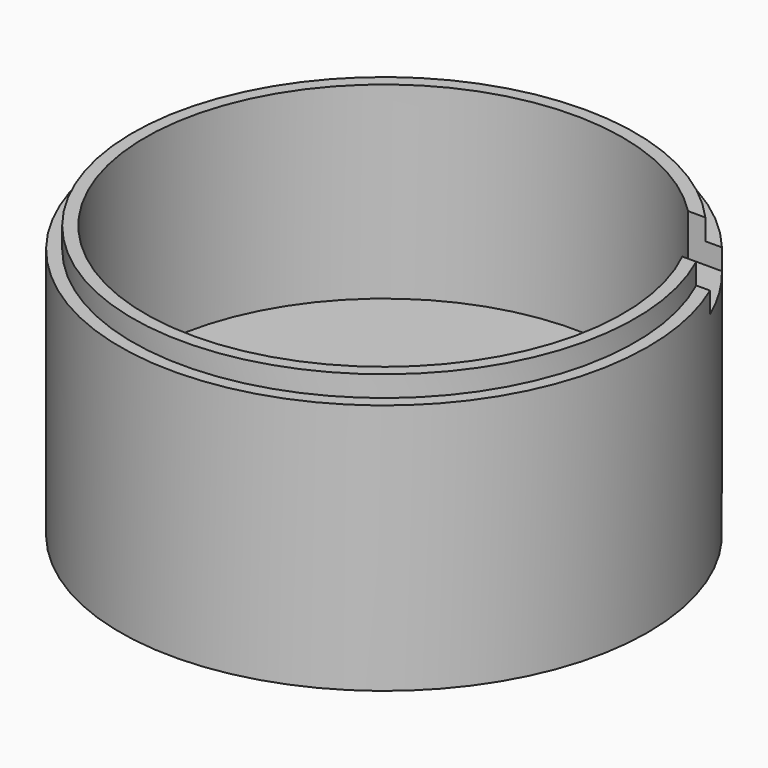
from build123d import *

# Parameters (mm, degrees)
F0_R      = 63
F0_R_2    = 60
F2_DEPTH  = 60
F1_R      = 60
F1_R_2    = 57
F3_DEPTH  = 65
F4_R      = 57
F5_DEPTH  = 60
F7_R      = 57
F8_DEPTH  = 40
F9_W      = 15
F9_H      = 10
F10_DEPTH = 279.5
F11_DEPTH = 71.5
F13_R     = 63
F14_DEPTH = 20
F15_W     = 86
F15_H     = 41
F16_DEPTH = 15
F18_DEPTH = 53
F20_DEPTH = 128


# Not quite as in the source:
# - a feature names something its author has since deleted; it is built from what else it names


with BuildPart() as f2:
    # F0 (on Top) → F2 (new body)
    with BuildSketch(Plane.XY):
        Circle(F0_R)
        Circle(F0_R_2, mode=Mode.SUBTRACT)
    extrude(amount=F2_DEPTH)

    # F1 (on Top) → F3 (join)
    with BuildSketch(Plane.XY):
        Circle(F1_R)
        Circle(F1_R_2, mode=Mode.SUBTRACT)
    extrude(amount=F3_DEPTH)

    # F4 (on Top) → F5 (join)
    with BuildSketch(Plane.XY):
        Circle(F4_R)
    extrude(amount=F5_DEPTH)

    # F7 (on offset) → F8 (cut)
    with BuildSketch(Plane.XY.offset(45)):
        Circle(F7_R)
    extrude(amount=-F8_DEPTH, mode=Mode.SUBTRACT)

    # F9 (on Right) → F10 (cut)
    with BuildSketch(Plane.YZ):
        with Locations((32.5, 60)):
            Rectangle(F9_W, F9_H)
    extrude(amount=F10_DEPTH, mode=Mode.SUBTRACT)

    # F1 (on Top) → F11 (cut)
    with BuildSketch(Plane.XY):
        Circle(F1_R_2)
    extrude(amount=F11_DEPTH, mode=Mode.SUBTRACT)

    # F13 (on Top) → F14 (join)
    with BuildSketch(Plane.XY):
        Circle(F13_R)
    extrude(amount=F14_DEPTH)

    # F15 (on Top) → F16 (cut)
    with BuildSketch(Plane.XY):
        Rectangle(F15_W, F15_H)
    extrude(amount=F16_DEPTH, mode=Mode.SUBTRACT)

    # F17 (on Right) → F18 (cut)
    with BuildSketch(Plane.YZ):
        Polygon((6.83, 15), (0, 15), (-20.47, 15), (-20.47, 2), (6.83, 2), align=None)
    extrude(amount=F18_DEPTH, mode=Mode.SUBTRACT)

    # F19 (on offset) → F20 (cut)
    with BuildSketch(Plane.XY.offset(15)):
        Polygon((43, 6.83), (43, 0), (43, -20.47), (53, -20.47), (53, 6.83), align=None)
    extrude(amount=F20_DEPTH, mode=Mode.SUBTRACT)


solid = f2.part
